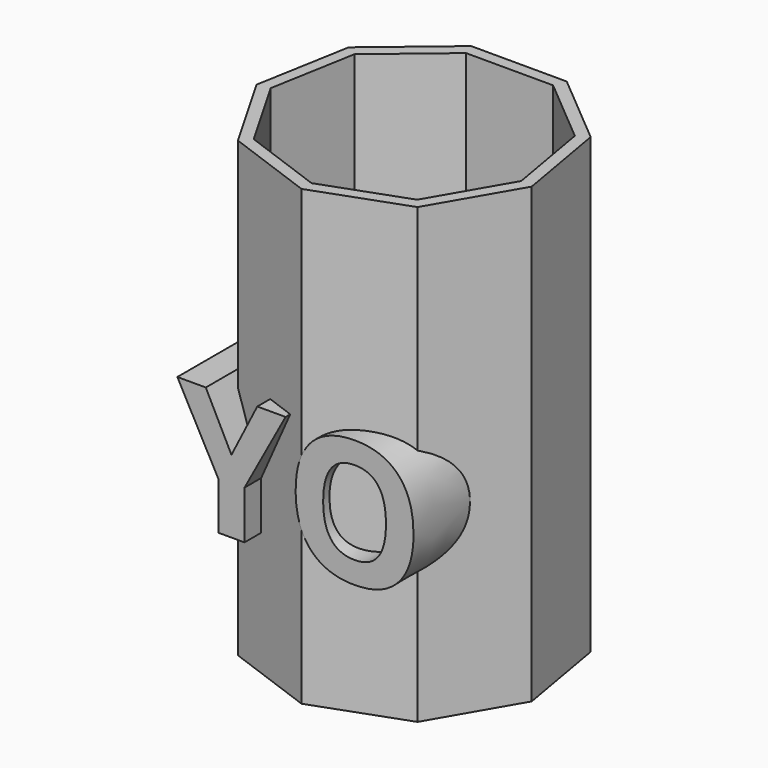
from build123d import *

# Parameters (mm, degrees)
F1_DEPTH     = 270
F2_T         = -7
F4_TEXT_SIZE = 103.3048662874


# Not quite as in the source:
# - Text() gives the source's letters only with a copy of the font that has no kerning and outlines rounded to 1/6400 em; it was checked with that copy


with BuildPart() as f1:
    # F0 (on Top) → F1 (new body)
    with BuildSketch(Plane.XY):
        Polygon((-28.3762846365, 78.3480245485), (-72.0986345853, 41.7781446614), (-82.0852321246, -14.3401934251), (-53.663237277, -63.7485956345), (-0.1316173071, -83.3283214598), (53.4615878636, -63.9177995829), (82.0395219136, -14.599428914), (72.2302518924, 41.5501767984), (28.623644261, 78.257993008), align=None)
    extrude(amount=F1_DEPTH)

    # F2
    f2_openings = [f1.faces().sort_by_distance(p)[0] for p in [
        (0, 0, 270),
    ]]
    offset(amount=F2_T, openings=f2_openings)

    # F4 (on offset) → F5 (join, up to the next surface of F1)
    with BuildSketch(Plane.XZ.offset(83.33)):
        with Locations((-74.0949958563, 73.5687315464)):
            Text('YO', F4_TEXT_SIZE, font='Open Sans', font_style=FontStyle.BOLD, text_align=(TextAlign.LEFT, TextAlign.BOTTOM))
    extrude(until=Until.NEXT, dir=(0, 1, 0))


solid = f1.part
